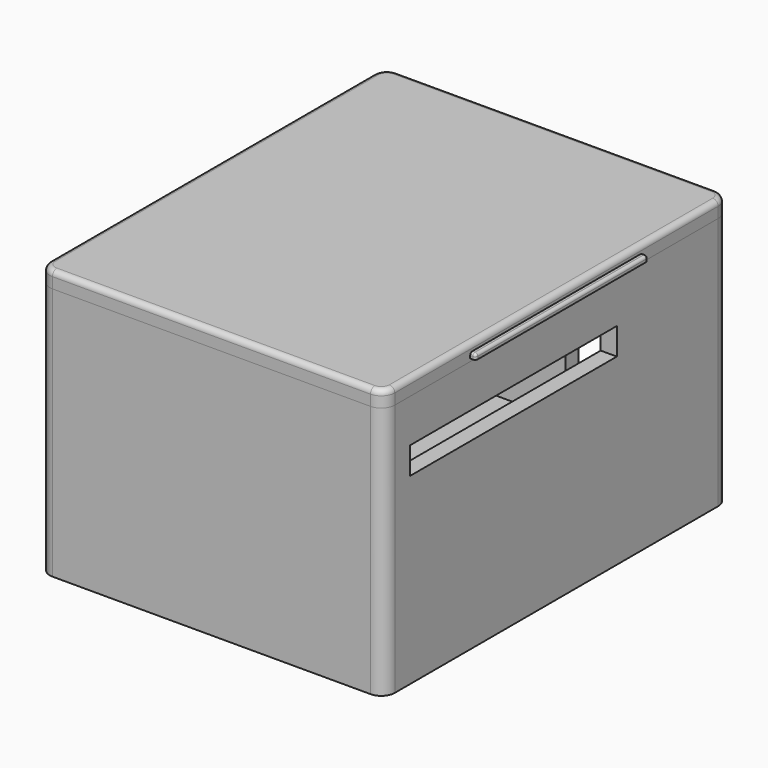
from build123d import *

# Parameters (mm, degrees)
F0_W            = 64
F0_H            = 80
F1_DEPTH        = 45
F2_T            = -3
F3_DEPTH        = 2
F4_W            = 64
F4_H            = 80
F4_W_2          = 58
F4_H_2          = 74
F4_W_3          = 56
F4_H_3          = 72
F5_DEPTH        = 3
F6_DEPTH        = 5
F7_R            = 2.7
F7_R_2          = 1.7
F8_DEPTH        = 5
F8_FACE_R       = 1.7
F7_R_3          = 1.6
F9_DEPTH        = 5
F10_R           = 1.7
F11_DEPTH       = 2.6
F12_W           = 14
F12_H           = 12.9
F12_W_2         = 10.9
F13_DEPTH       = 3
F14_W           = 48
F14_H           = 5
F15_DEPTH       = 3
F16_W           = 40
F16_H           = 1
F18_DEPTH       = 1
F17_W           = 40
F17_H           = 1
F19_DEPTH       = 1
F20_R           = 1
F21_R           = 0.5
F22_F1_R        = 2.5
F22_F2_R        = 2.5
F22_F3_R        = 2.5
F22_F4_R        = 2.5
F22_2_T1_DEPTH  = 3
F22_2_T4_ANGLE  = 90
F22_2_T6_ANGLE  = 90
F22_2_T8_ANGLE  = 90
F22_2_T10_ANGLE = 90


# Not quite as in the source:
# - a fillet or chamfer that OpenCascade refuses, or shapes differently, is made with other operations: its cross-section is extruded or revolved along the edge and cut away or added


with BuildPart() as f1:
    # F0 (on Top) → F1 (new body)
    with BuildSketch(Plane.XY):
        Rectangle(F0_W, F0_H)
    extrude(amount=F1_DEPTH)

    # F2
    f2_openings = [f1.faces().sort_by_distance(p)[0] for p in [
        (0, 0, 45),
    ]]
    offset(amount=F2_T, openings=f2_openings)

    # F3 (add): a face of the model
    f3_faces = [f1.faces().sort_by_distance(p)[0] for p in [
        (0, 0, 0),
    ]]
    extrude(f3_faces, amount=F3_DEPTH)

    # F7 (on face) → F8 (join)
    with BuildSketch(Plane.XY.offset(3)):
        with Locations((8.85, -30.9)):
            Circle(F7_R)
        with Locations((8.85, -30.9)):
            Circle(F7_R_2, mode=Mode.SUBTRACT)
        with Locations((-19.05, -30.9)):
            Circle(F7_R)
        with Locations((-19.05, -30.9)):
            Circle(F7_R_2, mode=Mode.SUBTRACT)
        with Locations((-24.15, 21.2)):
            Circle(F7_R)
        with Locations((-24.15, 21.2)):
            Circle(F7_R_2, mode=Mode.SUBTRACT)
        with Locations((24.05, 19.9)):
            Circle(F7_R)
        with Locations((24.05, 19.9)):
            Circle(F7_R_2, mode=Mode.SUBTRACT)
    extrude(amount=F8_DEPTH)

    # F8_face (on face) + F7 (on face) → F9 (cut)
    with BuildSketch(Plane(origin=(-24.15, 21.2, 3), x_dir=(1, 0, 0), z_dir=(0, 0, 1))):
        Circle(F8_FACE_R)
        with Locations((48.2, -1.3)):
            Circle(F8_FACE_R)
        with Locations((33, -52.1)):
            Circle(F8_FACE_R)
        with Locations((5.1, -52.1)):
            Circle(F8_FACE_R)
    with BuildSketch(Plane.XY.offset(3)):
        with Locations((-22.5, 30.5)):
            Circle(F7_R_3)
        with Locations((22.5, 30.5)):
            Circle(F7_R_3)
        with Locations((22.5, -20.5)):
            Circle(F7_R_3)
        with Locations((-22.5, -20.5)):
            Circle(F7_R_3)
    extrude(amount=-F9_DEPTH, mode=Mode.SUBTRACT)

    # F10 (on face) → F11 (cut)
    with BuildSketch(Plane(origin=(0, 0, -2), x_dir=(1, 0, 0), z_dir=(0, 0, -1))):
        with BuildLine():
            ThreePointArc((-16.6875000099, 29.5360099718), (-16.4149736458, 30.1939468061), (-16.3220199781, 30.9))
            ThreePointArc((-16.3220199781, 30.9), (-16.4149736458, 31.6060531939), (-16.6875000099, 32.2639900282))
            ThreePointArc((-16.6875000099, 32.2639900282), (-17.6860099976, 33.262500005), (-19.05, 33.6279800219))
            ThreePointArc((-19.05, 33.6279800219), (-20.4139900024, 33.262500005), (-21.4124999901, 32.2639900282))
            ThreePointArc((-21.4124999901, 32.2639900282), (-21.7779800219, 30.9), (-21.4124999901, 29.5360099718))
            ThreePointArc((-21.4124999901, 29.5360099718), (-20.4139900024, 28.537499995), (-19.05, 28.1720199781))
            ThreePointArc((-19.05, 28.1720199781), (-17.6860099976, 28.537499995), (-16.6875000099, 29.5360099718))
        make_face()
        with Locations((-19.05, 30.9)):
            Circle(F10_R, mode=Mode.SUBTRACT)
        with BuildLine():
            ThreePointArc((-16.6875000099, 32.2639900282), (-16.4149736458, 31.6060531939), (-16.3220199781, 30.9))
            ThreePointArc((-16.3220199781, 30.9), (-16.4149736458, 30.1939468061), (-16.6875000099, 29.5360099718))
            Line((-16.6875000099, 29.5360099718), (-15.9, 30.9))
            Line((-15.9, 30.9), (-16.6875000099, 32.2639900282))
        make_face()
        with BuildLine():
            ThreePointArc((-19.05, 33.6279800219), (-17.6860099976, 33.262500005), (-16.6875000099, 32.2639900282))
            Line((-16.6875000099, 32.2639900282), (-17.475, 33.6279800219))
            Line((-17.475, 33.6279800219), (-19.05, 33.6279800219))
        make_face()
        with BuildLine():
            Line((-17.475, 28.1720199781), (-16.6875000099, 29.5360099718))
            ThreePointArc((-16.6875000099, 29.5360099718), (-17.6860099976, 28.537499995), (-19.05, 28.1720199781))
            Line((-19.05, 28.1720199781), (-17.475, 28.1720199781))
        make_face()
        with BuildLine():
            ThreePointArc((-21.4124999901, 32.2639900282), (-20.4139900024, 33.262500005), (-19.05, 33.6279800219))
            Line((-19.05, 33.6279800219), (-20.625, 33.6279800219))
            Line((-20.625, 33.6279800219), (-21.4124999901, 32.2639900282))
        make_face()
        with BuildLine():
            Line((-20.625, 28.1720199781), (-19.05, 28.1720199781))
            ThreePointArc((-19.05, 28.1720199781), (-20.4139900024, 28.537499995), (-21.4124999901, 29.5360099718))
            Line((-21.4124999901, 29.5360099718), (-20.625, 28.1720199781))
        make_face()
        with BuildLine():
            ThreePointArc((-21.4124999901, 29.5360099718), (-21.7779800219, 30.9), (-21.4124999901, 32.2639900282))
            Line((-21.4124999901, 32.2639900282), (-22.2, 30.9))
            Line((-22.2, 30.9), (-21.4124999901, 29.5360099718))
        make_face()
        with BuildLine():
            ThreePointArc((11.2124999901, 29.5360099718), (11.4850263542, 30.1939468061), (11.5779800219, 30.9))
            ThreePointArc((11.5779800219, 30.9), (11.4850263637, 31.6060531587), (11.2125000266, 32.2639899649))
            ThreePointArc((11.2125000266, 32.2639899649), (10.213990034, 33.2624999867), (8.85, 33.6279800219))
            ThreePointArc((8.85, 33.6279800219), (7.486009993, 33.2625000023), (6.4875000046, 32.263990019))
            ThreePointArc((6.4875000046, 32.263990019), (6.1220199781, 30.9000000086), (6.487499996, 29.536009996))
            ThreePointArc((6.487499996, 29.536009996), (7.4860099856, 28.537500002), (8.85, 28.1720199781))
            ThreePointArc((8.85, 28.1720199781), (10.2139900024, 28.537499995), (11.2124999901, 29.5360099718))
        make_face()
        with Locations((8.85, 30.9)):
            Circle(F10_R, mode=Mode.SUBTRACT)
        with BuildLine():
            ThreePointArc((11.2125000266, 32.2639899649), (11.4850263637, 31.6060531587), (11.5779800219, 30.9))
            ThreePointArc((11.5779800219, 30.9), (11.4850263542, 30.1939468061), (11.2124999901, 29.5360099718))
            Line((11.2124999901, 29.5360099718), (12, 30.9))
            Line((12, 30.9), (11.2125000266, 32.2639899649))
        make_face()
        with BuildLine():
            ThreePointArc((8.85, 33.6279800219), (10.213990034, 33.2624999867), (11.2125000266, 32.2639899649))
            Line((11.2125000266, 32.2639899649), (10.425, 33.6279800219))
            Line((10.425, 33.6279800219), (8.85, 33.6279800219))
        make_face()
        with BuildLine():
            Line((10.425, 28.1720199781), (11.2124999901, 29.5360099718))
            ThreePointArc((11.2124999901, 29.5360099718), (10.2139900024, 28.537499995), (8.85, 28.1720199781))
            Line((8.85, 28.1720199781), (10.425, 28.1720199781))
        make_face()
        with BuildLine():
            ThreePointArc((6.4875000046, 32.263990019), (7.486009993, 33.2625000023), (8.85, 33.6279800219))
            Line((8.85, 33.6279800219), (7.275, 33.6279800219))
            Line((7.275, 33.6279800219), (6.4875000046, 32.263990019))
        make_face()
        with BuildLine():
            Line((7.275, 28.1720199781), (8.85, 28.1720199781))
            ThreePointArc((8.85, 28.1720199781), (7.4860099856, 28.537500002), (6.487499996, 29.536009996))
            Line((6.487499996, 29.536009996), (7.275, 28.1720199781))
        make_face()
        with BuildLine():
            ThreePointArc((6.487499996, 29.536009996), (6.1220199781, 30.9000000086), (6.4875000046, 32.263990019))
            Line((6.4875000046, 32.263990019), (5.7, 30.9))
            Line((5.7, 30.9), (6.487499996, 29.536009996))
        make_face()
        with BuildLine():
            ThreePointArc((-21.787500069, -22.5639901305), (-21.5149736611, -21.906053251), (-21.4220199781, -21.2))
            ThreePointArc((-21.4220199781, -21.2), (-21.5149736348, -20.4939468472), (-21.7874999673, -19.8360100456))
            ThreePointArc((-21.7874999673, -19.8360100456), (-22.7860099607, -18.8375000163), (-24.15, -18.4720199781))
            ThreePointArc((-24.15, -18.4720199781), (-25.5139900024, -18.837499995), (-26.5124999901, -19.8360099718))
            ThreePointArc((-26.5124999901, -19.8360099718), (-26.8779800219, -21.2), (-26.5124999901, -22.5639900282))
            ThreePointArc((-26.5124999901, -22.5639900282), (-25.5139900024, -23.562500005), (-24.15, -23.9279800219))
            ThreePointArc((-24.15, -23.9279800219), (-22.7860100488, -23.5625000345), (-21.787500069, -22.5639901305))
        make_face()
        with Locations((-24.15, -21.2)):
            Circle(F10_R, mode=Mode.SUBTRACT)
        with BuildLine():
            ThreePointArc((-21.7874999673, -19.8360100456), (-21.5149736348, -20.4939468472), (-21.4220199781, -21.2))
            ThreePointArc((-21.4220199781, -21.2), (-21.5149736611, -21.906053251), (-21.787500069, -22.5639901305))
            Line((-21.787500069, -22.5639901305), (-21, -21.2))
            Line((-21, -21.2), (-21.7874999673, -19.8360100456))
        make_face()
        with BuildLine():
            ThreePointArc((-24.15, -18.4720199781), (-22.7860099607, -18.8375000163), (-21.7874999673, -19.8360100456))
            Line((-21.7874999673, -19.8360100456), (-22.575, -18.4720199781))
            Line((-22.575, -18.4720199781), (-24.15, -18.4720199781))
        make_face()
        with BuildLine():
            Line((-22.575, -23.9279800219), (-21.787500069, -22.5639901305))
            ThreePointArc((-21.787500069, -22.5639901305), (-22.7860100488, -23.5625000345), (-24.15, -23.9279800219))
            Line((-24.15, -23.9279800219), (-22.575, -23.9279800219))
        make_face()
        with BuildLine():
            ThreePointArc((-26.5124999901, -19.8360099718), (-25.5139900024, -18.837499995), (-24.15, -18.4720199781))
            Line((-24.15, -18.4720199781), (-25.725, -18.4720199781))
            Line((-25.725, -18.4720199781), (-26.5124999901, -19.8360099718))
        make_face()
        with BuildLine():
            Line((-25.725, -23.9279800219), (-24.15, -23.9279800219))
            ThreePointArc((-24.15, -23.9279800219), (-25.5139900024, -23.562500005), (-26.5124999901, -22.5639900282))
            Line((-26.5124999901, -22.5639900282), (-25.725, -23.9279800219))
        make_face()
        with BuildLine():
            ThreePointArc((-26.5124999901, -22.5639900282), (-26.8779800219, -21.2), (-26.5124999901, -19.8360099718))
            Line((-26.5124999901, -19.8360099718), (-27.3, -21.2))
            Line((-27.3, -21.2), (-26.5124999901, -22.5639900282))
        make_face()
        with BuildLine():
            ThreePointArc((26.412499931, -21.2639901305), (26.6850263389, -20.606053251), (26.7779800219, -19.9))
            ThreePointArc((26.7779800219, -19.9), (26.6850263542, -19.1939468061), (26.4124999901, -18.5360099718))
            ThreePointArc((26.4124999901, -18.5360099718), (25.4139900024, -17.537499995), (24.05, -17.1720199781))
            ThreePointArc((24.05, -17.1720199781), (22.6860099804, -17.537500005), (21.68749999, -18.5360100063))
            ThreePointArc((21.68749999, -18.5360100063), (21.3220199781, -19.9000000199), (21.6875000099, -21.2639900282))
            ThreePointArc((21.6875000099, -21.2639900282), (22.6860099976, -22.262500005), (24.05, -22.6279800219))
            ThreePointArc((24.05, -22.6279800219), (25.4139899512, -22.2625000345), (26.412499931, -21.2639901305))
        make_face()
        with Locations((24.05, -19.9)):
            Circle(F10_R, mode=Mode.SUBTRACT)
        with BuildLine():
            ThreePointArc((26.4124999901, -18.5360099718), (26.6850263542, -19.1939468061), (26.7779800219, -19.9))
            ThreePointArc((26.7779800219, -19.9), (26.6850263389, -20.606053251), (26.412499931, -21.2639901305))
            Line((26.412499931, -21.2639901305), (27.2, -19.9))
            Line((27.2, -19.9), (26.4124999901, -18.5360099718))
        make_face()
        with BuildLine():
            ThreePointArc((24.05, -17.1720199781), (25.4139900024, -17.537499995), (26.4124999901, -18.5360099718))
            Line((26.4124999901, -18.5360099718), (25.625, -17.1720199781))
            Line((25.625, -17.1720199781), (24.05, -17.1720199781))
        make_face()
        with BuildLine():
            Line((25.625, -22.6279800219), (26.412499931, -21.2639901305))
            ThreePointArc((26.412499931, -21.2639901305), (25.4139899512, -22.2625000345), (24.05, -22.6279800219))
            Line((24.05, -22.6279800219), (25.625, -22.6279800219))
        make_face()
        with BuildLine():
            ThreePointArc((21.68749999, -18.5360100063), (22.6860099804, -17.537500005), (24.05, -17.1720199781))
            Line((24.05, -17.1720199781), (22.475, -17.1720199781))
            Line((22.475, -17.1720199781), (21.68749999, -18.5360100063))
        make_face()
        with BuildLine():
            Line((22.475, -22.6279800219), (24.05, -22.6279800219))
            ThreePointArc((24.05, -22.6279800219), (22.6860099976, -22.262500005), (21.6875000099, -21.2639900282))
            Line((21.6875000099, -21.2639900282), (22.475, -22.6279800219))
        make_face()
        with BuildLine():
            ThreePointArc((21.6875000099, -21.2639900282), (21.3220199781, -19.9000000199), (21.68749999, -18.5360100063))
            Line((21.68749999, -18.5360100063), (20.9, -19.9))
            Line((20.9, -19.9), (21.6875000099, -21.2639900282))
        make_face()
        with Locations((-19.05, 30.9)):
            Circle(F10_R)
        with Locations((8.85, 30.9)):
            Circle(F10_R)
        with Locations((-24.15, -21.2)):
            Circle(F10_R)
        with Locations((24.05, -19.9)):
            Circle(F10_R)
    extrude(amount=-F11_DEPTH, mode=Mode.SUBTRACT)

    # F12 (on face) → F13 (cut)
    with BuildSketch(Plane(origin=(0, 40, 0), x_dir=(-1, 0, 0), z_dir=(0, 1, 0))):
        with Locations((-11.05, 15.05)):
            Rectangle(F12_W, F12_H)
        with Locations((18.9, 15.05)):
            Rectangle(F12_W_2, F12_H)
    extrude(amount=-F13_DEPTH, mode=Mode.SUBTRACT)

    # F14 (on face) → F15 (cut)
    with BuildSketch(Plane.YZ.offset(32)):
        with Locations((-10, 34.5)):
            Rectangle(F14_W, F14_H)
    extrude(amount=-F15_DEPTH, mode=Mode.SUBTRACT)

    # F22: fillet of radius 2.5 on 4 edges, made by hand

    # F22_f1
    f22_f1_edges = [f1.edges().sort_by_distance(p)[0] for p in [
        (32, 40, 21.5),
    ]]
    fillet(f22_f1_edges, radius=F22_F1_R)

    # F22_f2
    f22_f2_edges = [f1.edges().sort_by_distance(p)[0] for p in [
        (-32, 40, 21.5),
    ]]
    fillet(f22_f2_edges, radius=F22_F2_R)

    # F22_f3
    f22_f3_edges = [f1.edges().sort_by_distance(p)[0] for p in [
        (32, -40, 21.5),
    ]]
    fillet(f22_f3_edges, radius=F22_F3_R)

    # F22_f4
    f22_f4_edges = [f1.edges().sort_by_distance(p)[0] for p in [
        (-32, -40, 21.5),
    ]]
    fillet(f22_f4_edges, radius=F22_F4_R)


with BuildPart() as f5:
    # F4 (on face) → F5 (new body)
    with BuildSketch(Plane.XY.offset(45)):
        Rectangle(F4_W, F4_H)
        Rectangle(F4_W_2, F4_H_2, mode=Mode.SUBTRACT)
        Rectangle(F4_W_2, F4_H_2)
        Rectangle(F4_W_3, F4_H_3, mode=Mode.SUBTRACT)
        Rectangle(F4_W_3, F4_H_3)
    extrude(amount=F5_DEPTH)

    # F4 (on face) → F6 (join)
    with BuildSketch(Plane.XY.offset(45)):
        Rectangle(F4_W_3, F4_H_3)
    extrude(amount=-F6_DEPTH)

    # F16 (on face) → F18 (join)
    with BuildSketch(Plane.YZ.offset(32)):
        with Locations((0, 46)):
            Rectangle(F16_W, F16_H)
    extrude(amount=F18_DEPTH)

    # F17 (on face) → F19 (join)
    with BuildSketch(Plane(origin=(-32, 0, 0), x_dir=(0, -1, 0), z_dir=(-1, 0, 0))):
        with Locations((0, 46)):
            Rectangle(F17_W, F17_H)
    extrude(amount=F19_DEPTH)

    # F20
    f20_edges = [f5.edges().sort_by_distance(p)[0] for p in [
        (32, 0, 48),
        (0, -40, 48),
        (-32, 0, 48),
        (0, 40, 48),
    ]]
    fillet(f20_edges, radius=F20_R)

    # F21
    f21_edges = [f5.edges().sort_by_distance(p)[0] for p in [
        (-33, 0, 46.5),
        (-32.5, 20, 46.5),
        (-32.5, -20, 46.5),
        (32.5, -20, 46.5),
        (33, 0, 46.5),
        (32.5, 20, 46.5),
        (-33, 20, 46),
        (-33, -20, 46),
        (33, -20, 46),
        (33, 20, 46),
    ]]
    fillet(f21_edges, radius=F21_R)

    # F22#2: fillet of radius 2.5 on 4 edges, made by hand

    # F22_2_s2 → F22_2_t1 (cut)
    with BuildSketch(Plane.XY.offset(45)):
        with BuildLine():
            ThreePointArc((32, -37.5), (31.267766953, -39.267766953), (29.5, -40))
            Line((29.5, -40), (29.5, -40.05))
            Line((29.5, -40.05), (32.05, -40.05))
            Line((32.05, -40.05), (32.05, -37.5))
            Line((32.05, -37.5), (32, -37.5))
        make_face()
        with BuildLine():
            ThreePointArc((-29.5, -40), (-31.267766953, -39.267766953), (-32, -37.5))
            Line((-32, -37.5), (-32.05, -37.5))
            Line((-32.05, -37.5), (-32.05, -40.05))
            Line((-32.05, -40.05), (-29.5, -40.05))
            Line((-29.5, -40.05), (-29.5, -40))
        make_face()
        with BuildLine():
            ThreePointArc((32, 37.5), (31.267766953, 39.267766953), (29.5, 40))
            Line((29.5, 40), (29.5, 40.05))
            Line((29.5, 40.05), (32.05, 40.05))
            Line((32.05, 40.05), (32.05, 37.5))
            Line((32.05, 37.5), (32, 37.5))
        make_face()
        with BuildLine():
            ThreePointArc((-29.5, 40), (-31.267766953, 39.267766953), (-32, 37.5))
            Line((-32, 37.5), (-32.05, 37.5))
            Line((-32.05, 37.5), (-32.05, 40.05))
            Line((-32.05, 40.05), (-29.5, 40.05))
            Line((-29.5, 40.05), (-29.5, 40))
        make_face()
    extrude(amount=F22_2_T1_DEPTH, mode=Mode.SUBTRACT)

    # F22_2_s3 → F22_2_t4 (revolve, cut)
    with BuildSketch(Plane.YZ.offset(-29.5)):
        with BuildLine():
            ThreePointArc((39, 48), (39.7071067812, 47.7071067812), (40, 47))
            Line((40, 47), (40, 48))
            Line((40, 48), (39, 48))
        make_face()
    revolve(axis=Axis((-29.5, 37.5, 48), (0, 0, 1)), revolution_arc=F22_2_T4_ANGLE, mode=Mode.SUBTRACT)

    # F22_2_s5 → F22_2_t6 (revolve, cut)
    with BuildSketch(Plane.XZ.offset(-37.5)):
        with BuildLine():
            ThreePointArc((31, 48), (31.7071067812, 47.7071067812), (32, 47))
            Line((32, 47), (32, 48))
            Line((32, 48), (31, 48))
        make_face()
    revolve(axis=Axis((29.5, 37.5, 48), (0, 0, 1)), revolution_arc=F22_2_T6_ANGLE, mode=Mode.SUBTRACT)

    # F22_2_s7 → F22_2_t8 (revolve, cut)
    with BuildSketch(Plane.XZ.offset(37.5)):
        with BuildLine():
            ThreePointArc((-31, 48), (-31.7071067812, 47.7071067812), (-32, 47))
            Line((-32, 47), (-32, 48))
            Line((-32, 48), (-31, 48))
        make_face()
    revolve(axis=Axis((-29.5, -37.5, 48), (0, 0, 1)), revolution_arc=F22_2_T8_ANGLE, mode=Mode.SUBTRACT)

    # F22_2_s9 → F22_2_t10 (revolve, cut)
    with BuildSketch(Plane.YZ.offset(29.5)):
        with BuildLine():
            ThreePointArc((-39, 48), (-39.7071067812, 47.7071067812), (-40, 47))
            Line((-40, 47), (-40, 48))
            Line((-40, 48), (-39, 48))
        make_face()
    revolve(axis=Axis((29.5, -37.5, 48), (0, 0, 1)), revolution_arc=F22_2_T10_ANGLE, mode=Mode.SUBTRACT)


solid = Compound([f1.part, f5.part])
